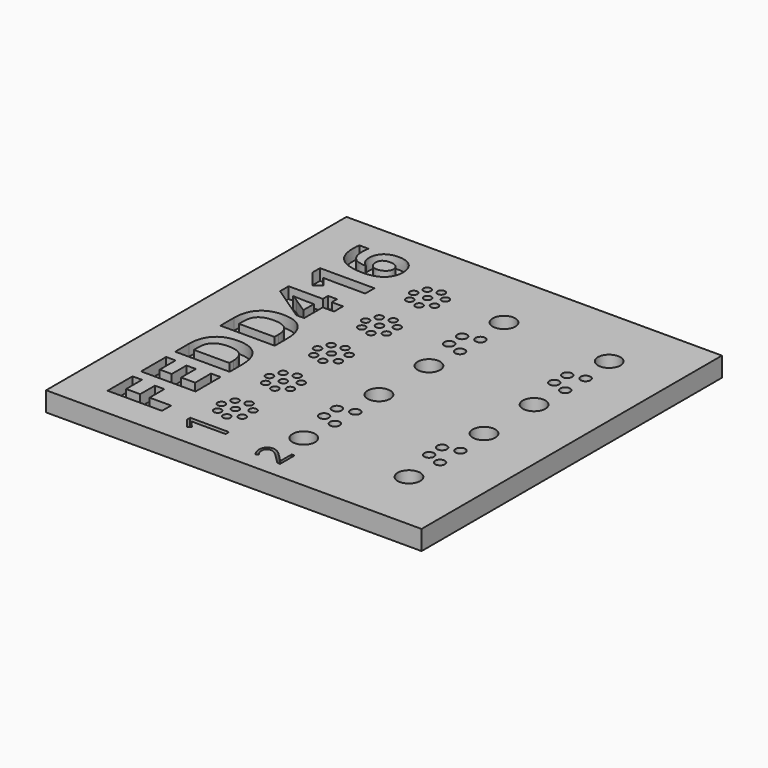
from build123d import *

# Parameters (mm, degrees)
F0_W           = 50
F0_H           = 50
F1_DEPTH       = 2.6
F2_TEXT_SIZE   = 10.1499423299
F2_TEXT_SIZE_2 = 7.24801812
F2_TEXT_SIZE_3 = 5.1460734388
F3_DEPTH       = 1.5
F4_R           = 0.5
F4_R_2         = 1.5
F4_R_3         = 0.65
F5_DEPTH       = 2.6


# Not quite as in the source:
# - Text() gives the source's letters only with a copy of the font that has no kerning and outlines rounded to 1/6400 em; it was checked with that copy


with BuildPart() as f1:
    # F0 (on Top) → F1 (new body)
    with BuildSketch(Plane.XY):
        with Locations((-18.1587231159, 3.3350909071)):
            Rectangle(F0_W, F0_H)
    extrude(amount=F1_DEPTH)

    # F2 (on face) → F3 (cut)
    with BuildSketch(Plane.XY.offset(2.6)):
        with Locations(Location((-30.8507646384, -18.6649090929), (0, 0, 90))):
            Text('FEDD416', F2_TEXT_SIZE, font='Open Sans', font_style=FontStyle.BOLD, text_align=(TextAlign.LEFT, TextAlign.BOTTOM))
        with Locations(Location((-22.41861649, -19.6649090929), (0, 0, 90))):
            Text('1', F2_TEXT_SIZE_2, font='Open Sans', text_align=(TextAlign.LEFT, TextAlign.BOTTOM))
        with Locations(Location((-13.7982989309, -19.6649041027), (0, 0, 90))):
            Text('2', F2_TEXT_SIZE_3, font='Open Sans', text_align=(TextAlign.LEFT, TextAlign.BOTTOM))
    extrude(amount=-F3_DEPTH, mode=Mode.SUBTRACT)

    # F4 (on face) → F5 (cut, through all)
    with BuildSketch(Plane.XY.offset(2.6)):
        with Locations((-27.0087231159, -4.6649090929)):
            Circle(F4_R)
        with Locations((-25.1587231159, -4.6649090929)):
            Circle(F4_R)
        with Locations((-26.3587231159, -3.2149090929)):
            Circle(F4_R)
        with Locations((-24.8087231159, -2.8149090929)):
            Circle(F4_R)
        with Locations((-23.5087231159, -3.7649090929)):
            Circle(F4_R)
        with Locations((-23.5087231159, -5.5649090929)):
            Circle(F4_R)
        with Locations((-24.8087231159, -6.5149090929)):
            Circle(F4_R)
        with Locations((-26.3587231159, -6.1149090929)):
            Circle(F4_R)
        with Locations((-27.0087231159, 3.3350909071)):
            Circle(F4_R)
        with Locations((-25.1587231159, 3.3350909071)):
            Circle(F4_R)
        with Locations((-26.3587231159, 4.7850909071)):
            Circle(F4_R)
        with Locations((-24.8087231159, 5.1850909071)):
            Circle(F4_R)
        with Locations((-23.5087231159, 4.2350909071)):
            Circle(F4_R)
        with Locations((-23.5087231159, 2.4350909071)):
            Circle(F4_R)
        with Locations((-24.8087231159, 1.4850909071)):
            Circle(F4_R)
        with Locations((-26.3587231159, 1.8850909071)):
            Circle(F4_R)
        with Locations((-27.0087231159, -12.6649090929)):
            Circle(F4_R)
        with Locations((-25.1587231159, -12.6649090929)):
            Circle(F4_R)
        with Locations((-26.3587231159, -11.2149090929)):
            Circle(F4_R)
        with Locations((-24.8087231159, -10.8149090929)):
            Circle(F4_R)
        with Locations((-23.5087231159, -11.7649090929)):
            Circle(F4_R)
        with Locations((-23.5087231159, -13.5649090929)):
            Circle(F4_R)
        with Locations((-24.8087231159, -14.5149090929)):
            Circle(F4_R)
        with Locations((-26.3587231159, -14.1149090929)):
            Circle(F4_R)
        with Locations((-27.0087231159, 11.3350909071)):
            Circle(F4_R)
        with Locations((-25.1587231159, 11.3350909071)):
            Circle(F4_R)
        with Locations((-26.3587231159, 12.7850909071)):
            Circle(F4_R)
        with Locations((-24.8087231159, 13.1850909071)):
            Circle(F4_R)
        with Locations((-23.5087231159, 12.2350909071)):
            Circle(F4_R)
        with Locations((-23.5087231159, 10.4350909071)):
            Circle(F4_R)
        with Locations((-24.8087231159, 9.4850909071)):
            Circle(F4_R)
        with Locations((-26.3587231159, 9.8850909071)):
            Circle(F4_R)
        with Locations((-27.0087231159, 19.3350909071)):
            Circle(F4_R)
        with Locations((-25.1587231159, 19.3350909071)):
            Circle(F4_R)
        with Locations((-26.3587231159, 20.7850909071)):
            Circle(F4_R)
        with Locations((-24.8087231159, 21.1850909071)):
            Circle(F4_R)
        with Locations((-23.5087231159, 20.2350909071)):
            Circle(F4_R)
        with Locations((-23.5087231159, 18.4350909071)):
            Circle(F4_R)
        with Locations((-24.8087231159, 17.4850909071)):
            Circle(F4_R)
        with Locations((-26.3587231159, 17.8850909071)):
            Circle(F4_R)
        with Locations((-15.5087231159, -13.3249090929)):
            Circle(F4_R_2)
        with Locations((-15.5087231159, -0.8249090929)):
            Circle(F4_R_2)
        with Locations((-15.0087231159, -8.7749090929)):
            Circle(F4_R_3)
        with Locations((-15.0087231159, -5.3749090929)):
            Circle(F4_R_3)
        with Locations((-16.9587231159, -8.1499090929)):
            Circle(F4_R_3)
        with Locations((-16.9587231159, -5.9999090929)):
            Circle(F4_R_3)
        with Locations((-15.5087231159, 7.5050909071)):
            Circle(F4_R_2)
        with Locations((-15.5087231159, 20.0050909071)):
            Circle(F4_R_2)
        with Locations((-15.0087231159, 12.0550909071)):
            Circle(F4_R_3)
        with Locations((-15.0087231159, 15.4550909071)):
            Circle(F4_R_3)
        with Locations((-16.9587231159, 12.6800909071)):
            Circle(F4_R_3)
        with Locations((-16.9587231159, 14.8300909071)):
            Circle(F4_R_3)
        with Locations((-1.5087231159, -13.3249090929)):
            Circle(F4_R_2)
        with Locations((-1.5087231159, -0.8249090929)):
            Circle(F4_R_2)
        with Locations((-1.0087231159, -8.7749090929)):
            Circle(F4_R_3)
        with Locations((-1.0087231159, -5.3749090929)):
            Circle(F4_R_3)
        with Locations((-2.9587231159, -8.1499090929)):
            Circle(F4_R_3)
        with Locations((-2.9587231159, -5.9999090929)):
            Circle(F4_R_3)
        with Locations((-1.5087231159, 7.5050909071)):
            Circle(F4_R_2)
        with Locations((-1.5087231159, 20.0050909071)):
            Circle(F4_R_2)
        with Locations((-1.0087231159, 12.0550909071)):
            Circle(F4_R_3)
        with Locations((-1.0087231159, 15.4550909071)):
            Circle(F4_R_3)
        with Locations((-2.9587231159, 12.6800909071)):
            Circle(F4_R_3)
        with Locations((-2.9587231159, 14.8300909071)):
            Circle(F4_R_3)
    extrude(amount=-F5_DEPTH, mode=Mode.SUBTRACT)


solid = f1.part
